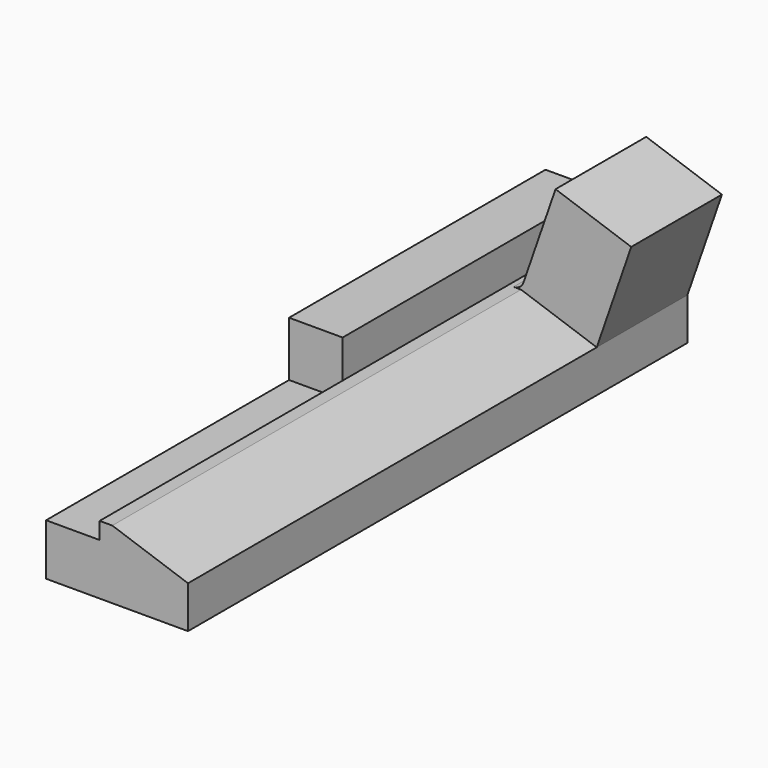
from build123d import *

# Parameters (mm, degrees)
F1_DEPTH = 288
F3_DEPTH = 304
F5_W     = 50.8
F5_H     = 304
F6_DEPTH = 36
F7_W     = 75.9582033121
F7_H     = 107.4988492727
F8_DEPTH = 100
F9_R     = 10


with BuildPart() as f1:
    # F0 (on Front) → F1 (new body)
    with BuildSketch(Plane.XZ):
        Polygon((0, 48.8444454968), (0, 0), (134.5802352905, 0), (134.5802352905, 40), (62.8, 64.8444454968), (50.8, 64.8444454968), (50.8, 48.8444454968), align=None)
    extrude(amount=F1_DEPTH)

    # F2 (on Front) → F3 (join)
    with BuildSketch(Plane.XZ):
        Polygon((0, 0), (134.5802352905, 0), (134.5802352905, 40), (62.8, 64.8444454968), (0, 64.8444454968), align=None)
    extrude(amount=-F3_DEPTH)

    # F5 (on face) → F6 (join)
    with BuildSketch(Plane.XY.offset(64.8444454968)):
        with Locations((25.4, 152)):
            Rectangle(F5_W, F5_H)
    extrude(amount=F6_DEPTH)

    # F7 (on face) → F8 (join)
    with BuildSketch(Plane(origin=(26.7612103496, 0, 77.3181263313), x_dir=(0.944996487, 0, -0.3270804787), z_dir=(0.3270804787, 0, 0.944996487))):
        with Locations((76.1155287701, 250.2505753636)):
            Rectangle(F7_W, F7_H)
    extrude(amount=F8_DEPTH)

    # F9
    f9_edges = [f1.edges().sort_by_distance(p)[0] for p in [
        (62.8, 250.250575, 64.844445),
    ]]
    fillet(f9_edges, radius=F9_R)


solid = f1.part
